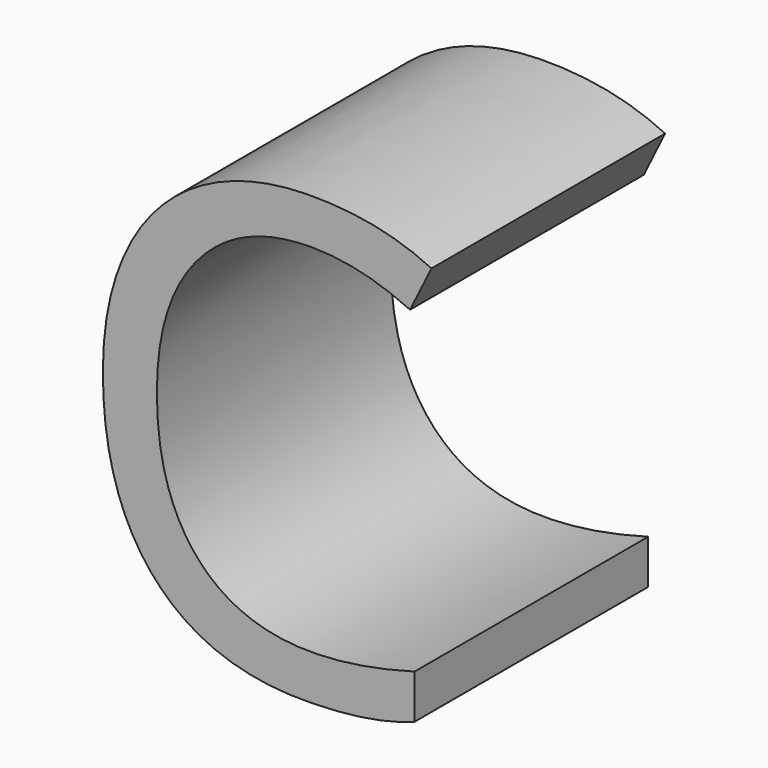
from build123d import *

# Parameters (mm, degrees)
F0_TEXT_SIZE = 52.9166666667
F1_DEPTH     = 25.4


# Not quite as in the source:
# - Text() gives the source's letters only with a copy of the font that has no kerning and outlines rounded to 1/6400 em; it was checked with that copy


with BuildPart() as f1:
    # F0 (on Front) → F1 (new body)
    with BuildSketch(Plane.XZ):
        with Locations((-14.5801684649, -19.9013970407)):
            Text('C', F0_TEXT_SIZE, font='Open Sans', text_align=(TextAlign.LEFT, TextAlign.BOTTOM))
    extrude(amount=F1_DEPTH)


solid = f1.part
